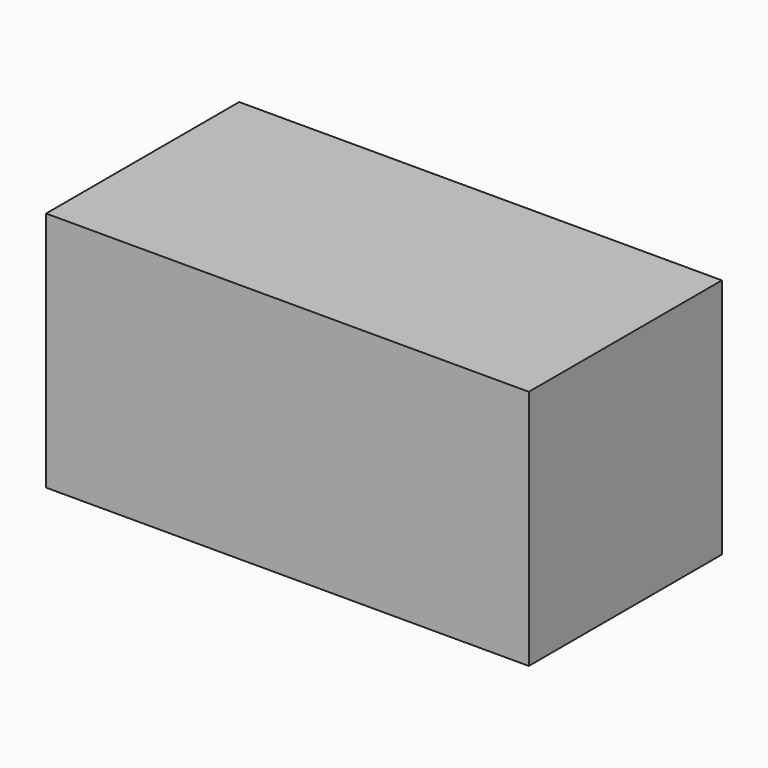
from build123d import *

# Parameters (mm, degrees)
F1_W      = 30560
F1_H      = 15280
F2_DEPTH  = 140
F3_W      = 30560
F3_H      = 15280
F3_W_2    = 15000
F3_H_2    = 15000
F4_DEPTH  = 6850
F5_W      = 30560
F5_H      = 15280
F6_DEPTH  = 1300
F10_W     = 30560
F10_H     = 15280
F10_W_2   = 280
F10_H_2   = 1300
F11_DEPTH = 6850
F12_DEPTH = 280
F13_W     = 30560
F13_H     = 15280
F13_W_2   = 15000
F13_H_2   = 15000
F14_DEPTH = 140


with BuildPart() as f2:
    # F1 (on offset) → F2 (new body)
    with BuildSketch(Plane.XY.offset(-15140)):
        Rectangle(F1_W, F1_H)
    extrude(amount=F2_DEPTH)

    # F3 (on face) → F4 (join)
    with BuildSketch(Plane.XY.offset(-15000)):
        Rectangle(F3_W, F3_H)
        with Locations((-7640, 0)):
            Rectangle(F3_W_2, F3_H_2, mode=Mode.SUBTRACT)
        with Locations((7640, 0)):
            Rectangle(F3_W_2, F3_H_2, mode=Mode.SUBTRACT)
    extrude(amount=F4_DEPTH)

    # F5 (on face) → F6 (join)
    with BuildSketch(Plane.XY.offset(-8150)):
        Rectangle(F5_W, F5_H)
        Polygon((-15140, -7500), (-15140, 7500), (-140, 7500), (-140, 650), (140, 650), (140, 7500), (15140, 7500), (15140, -7500), (140, -7500), (140, -650), (-140, -650), (-140, -7500), align=None, mode=Mode.SUBTRACT)
    extrude(amount=F6_DEPTH)

    # F10 (on face) → F11 (join)
    with BuildSketch(Plane.XY.offset(-6850)):
        Rectangle(F10_W, F10_H)
        Polygon((-15140, -7500), (-15140, 7500), (-140, 7500), (-140, 650), (140, 650), (140, 7500), (15140, 7500), (15140, -7500), (140, -7500), (140, -650), (-140, -650), (-140, -7500), align=None, mode=Mode.SUBTRACT)
        Rectangle(F10_W_2, F10_H_2)
    extrude(amount=F11_DEPTH)

    # F9 (on face) → F12 (join)
    with BuildSketch(Plane(origin=(-140, 0, 0), x_dir=(0, -1, 0), z_dir=(-1, 0, 0))):
        with BuildLine():
            Line((650, -7500), (650, -6850))
            Line((650, -6850), (6.2463e-06, -6850))
            ThreePointArc((6.2463e-06, -6850), (459.6194099796, -7040.3805944371), (650, -7500))
        make_face()
        with BuildLine():
            ThreePointArc((-650, -7500), (-459.6194055629, -7040.3805900204), (6.2463e-06, -6850))
            Line((6.2463e-06, -6850), (-650, -6850))
            Line((-650, -6850), (-650, -7500))
        make_face()
        with BuildLine():
            Line((650, -8150), (650, -7500))
            ThreePointArc((650, -7500), (459.6194077131, -7959.6194078294), (-1.644e-07, -8150))
            Line((-1.644e-07, -8150), (650, -8150))
        make_face()
        with BuildLine():
            ThreePointArc((-1.644e-07, -8150), (-459.6194078294, -7959.6194077131), (-650, -7500))
            Line((-650, -7500), (-650, -8150))
            Line((-650, -8150), (-1.644e-07, -8150))
        make_face()
    extrude(amount=-F12_DEPTH)

    # F13 (on face) → F14 (join)
    with BuildSketch(Plane.XY):
        Rectangle(F13_W, F13_H)
        with Locations((-7640, 0)):
            Rectangle(F13_W_2, F13_H_2, mode=Mode.SUBTRACT)
        with Locations((7640, 0)):
            Rectangle(F13_W_2, F13_H_2, mode=Mode.SUBTRACT)
        with Locations((-7640, 0)):
            Rectangle(F13_W_2, F13_H_2)
        with Locations((7640, 0)):
            Rectangle(F13_W_2, F13_H_2)
    extrude(amount=F14_DEPTH)


solid = f2.part
